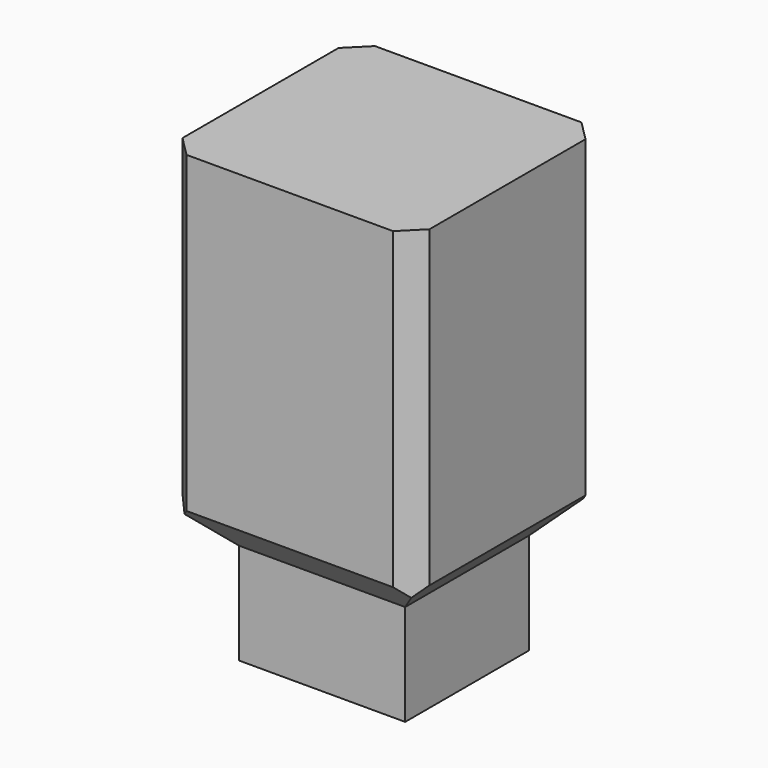
from build123d import *

# Parameters (mm, degrees)
F0_W     = 62.0293021202
F0_H     = 59.1503232718
F1_DEPTH = 88.9
F2_W     = 40.0586724281
F2_H     = 35.1866781712
F3_DEPTH = 76.2
F4_SIZE  = 5.08
F5_SIZE  = 10.16
F6_T     = 2.54
F7_DEPTH = 25.4


# Not quite as in the source:
# - a shell that OpenCascade refuses in one call is made with other operations: the cavity is built on its own and cut out


with BuildPart() as f1:
    # F0 (on Top) → F1 (new body)
    with BuildSketch(Plane.XY):
        with Locations((0.0738501549, -1.0445043445)):
            Rectangle(F0_W, F0_H)
    extrude(amount=-F1_DEPTH)

    # F2 (on face) → F3 (cut, symmetric)
    with BuildSketch(Plane(origin=(0, 0, -88.9), x_dir=(1, 0, 0), z_dir=(0, 0, -1))):
        with Locations((-0.360891223, -0.2706944942)):
            Rectangle(F2_W, F2_H)
    extrude(amount=F3_DEPTH, both=True, mode=Mode.SUBTRACT)

    # F4
    f4_edges = [f1.edges().sort_by_distance(p)[0] for p in [
        (-30.940801, 28.530657, -44.45),
        (31.088501, 28.530657, -44.45),
        (31.088501, -30.619666, -44.45),
        (-30.940801, -30.619666, -44.45),
    ]]
    chamfer(f4_edges, length=F4_SIZE)

    # F5 (call 1 of 4: OpenCascade refuses the feature's edges together)
    f5_edges = [f1.edges().sort_by_distance(p)[0] for p in [
        (0.07385, -30.619666, -88.9),
    ]]
    chamfer(f5_edges, length=F5_SIZE)

    # F5#2 (call 2 of 4)
    f5_2_edges = [f1.edges().sort_by_distance(p)[0] for p in [
        (0.07385, 28.530657, -88.9),
    ]]
    chamfer(f5_2_edges, length=F5_SIZE)

    # F5#3 (call 3 of 4)
    f5_3_edges = [f1.edges().sort_by_distance(p)[0] for p in [
        (31.088501, -1.044504, -88.9),
    ]]
    chamfer(f5_3_edges, length=F5_SIZE)

    # F5#4 (call 4 of 4)
    f5_4_edges = [f1.edges().sort_by_distance(p)[0] for p in [
        (-30.940801, -1.044504, -88.9),
    ]]
    chamfer(f5_4_edges, length=F5_SIZE)

    # F6: shell of thickness 2.54, made by hand


with BuildPart() as f6_core1:
    # F6_t2: copy of F1
    add(f1.part)

    # the walls: a layer under each face that stays
    f6_faces = [f6_core1.faces().sort_by_distance(p)[0] for p in [
        (0.0738501549, 23.4506572914, -83.82),
        (-17.8015650395, -17.6860714609, -88.9),
        (-25.8608009052, -1.0445043445, -83.82),
        (26.008501215, -1.0445043445, -83.82),
        (-28.4008009052, 25.9906572914, -40.64),
        (28.548501215, 25.9906572914, -40.64),
        (0.0738501549, 28.5306572914, -39.37),
        (0.0738501549, -25.5396659803, -83.82),
        (-30.9408009052, -1.0445043445, -39.37),
        (-28.4008009052, -28.0796659803, -40.64),
        (28.548501215, -28.0796659803, -40.64),
        (31.088501215, -1.0445043445, -39.37),
        (0.0738501549, -1.0445043445, 0),
        (0.0738501549, -30.6196659803, -39.37),
    ]]
    thicken(f6_faces, amount=-F6_T, mode=Mode.SUBTRACT)


with BuildPart() as f1_1:
    add(f1.part)

    # what is left inside the walls is the cavity
    f6_cavity = [f6_core1.part.solids().sort_by_distance(p)[0] for p in [
        (0.07385, 25.965257, -52.638598),
    ]]
    add(f6_cavity, mode=Mode.SUBTRACT)

    # F7 (add): a face of the model
    f7_faces = [f1_1.faces().sort_by_distance(p)[0] for p in [
        (0.0738501549, 18.3136708028, -88.9),
    ]]
    extrude(f7_faces, amount=F7_DEPTH)


solid = f1_1.part
